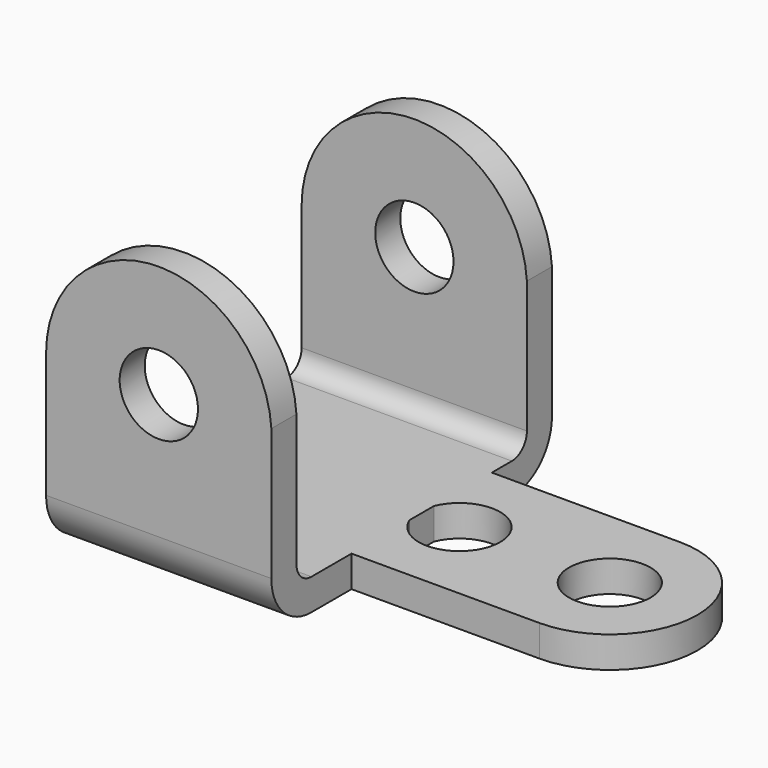
from build123d import *

# Parameters (mm, degrees)
F0_R     = 10.3251
F1_DEPTH = 7.9375
F3_DEPTH = 57.0992
F4_R     = 9.92251
F5_DEPTH = 88.901
F7_DEPTH = 127.001


with BuildPart() as f1:
    # F0 (on Top) → F1 (new body)
    with BuildSketch(Plane.XY):
        with BuildLine():
            Line((0, 88.9), (0, 0))
            Line((0, 0), (50.8, 0))
            Line((50.8, 0), (50.8, 19.05))
            ThreePointArc((50.8, 19.05), (52.6598719395, 23.5401280605), (57.15, 25.4))
            Line((57.15, 25.4), (104.775, 25.4))
            ThreePointArc((104.775, 25.4), (127, 47.625), (104.775, 69.85))
            Line((104.775, 69.85), (57.15, 69.85))
            ThreePointArc((57.15, 69.85), (52.6598719395, 71.7098719395), (50.8, 76.2))
            Line((50.8, 76.2), (50.8, 88.9))
            Line((50.8, 88.9), (0, 88.9))
        make_face()
        with Locations((66.675, 47.625)):
            Circle(F0_R, mode=Mode.SUBTRACT)
        with Locations((104.775, 47.625)):
            Circle(F0_R, mode=Mode.SUBTRACT)
    extrude(amount=F1_DEPTH)

    # F2 (on Right) → F3 (join)
    with BuildSketch(Plane.YZ):
        with BuildLine():
            Line((0, 76.2), (0, 12.7))
            ThreePointArc((0, 12.7), (3.7197438789, 3.7197438789), (12.7, 0))
            Line((12.7, 0), (76.2, 0))
            ThreePointArc((76.2, 0), (85.1802561211, 3.7197438789), (88.9, 12.7))
            Line((88.9, 12.7), (88.9, 76.2))
            Line((88.9, 76.2), (80.9625, 76.2))
            Line((80.9625, 76.2), (80.9625, 12.7))
            ThreePointArc((80.9625, 12.7), (79.5675960454, 9.3324039546), (76.2, 7.9375))
            Line((76.2, 7.9375), (12.7, 7.9375))
            ThreePointArc((12.7, 7.9375), (9.3324039546, 9.3324039546), (7.9375, 12.7))
            Line((7.9375, 12.7), (7.9375, 76.2))
            Line((7.9375, 76.2), (0, 76.2))
        make_face()
    extrude(amount=F3_DEPTH)

    # F4 (on Front) → F5 (cut, through all)
    with BuildSketch(Plane.XZ):
        with Locations((28.575, 44.45)):
            Circle(F4_R)
        with BuildLine():
            Line((57.1075950167, 46.0061640709), (57.1084559489, 42.9097024275))
            ThreePointArc((57.1084559489, 42.9097024275), (57.1499988955, 44.4579449194), (57.1075950167, 46.0061640709))
        make_face()
        with BuildLine():
            ThreePointArc((0, 44.45), (27.7966291375, 73.0143967869), (57.1075950167, 46.0061640709))
            Line((57.1075950167, 46.0061640709), (57.0992, 76.2))
            Line((57.0992, 76.2), (0, 76.2))
            Line((0, 76.2), (0, 44.45))
        make_face()
    extrude(amount=-F5_DEPTH, mode=Mode.SUBTRACT)

    # F6 (on Right) → F7 (cut, through all)
    with BuildSketch(Plane.YZ):
        with BuildLine():
            Line((0, 12.7), (0, 0))
            Line((0, 0), (12.7, 0))
            ThreePointArc((12.7, 0), (3.7197438789, 3.7197438789), (0, 12.7))
        make_face()
        with BuildLine():
            Line((76.2, 0), (88.9, 0))
            Line((88.9, 0), (88.9, 12.7))
            ThreePointArc((88.9, 12.7), (85.1802561211, 3.7197438789), (76.2, 0))
        make_face()
    extrude(amount=F7_DEPTH, mode=Mode.SUBTRACT)


solid = f1.part
